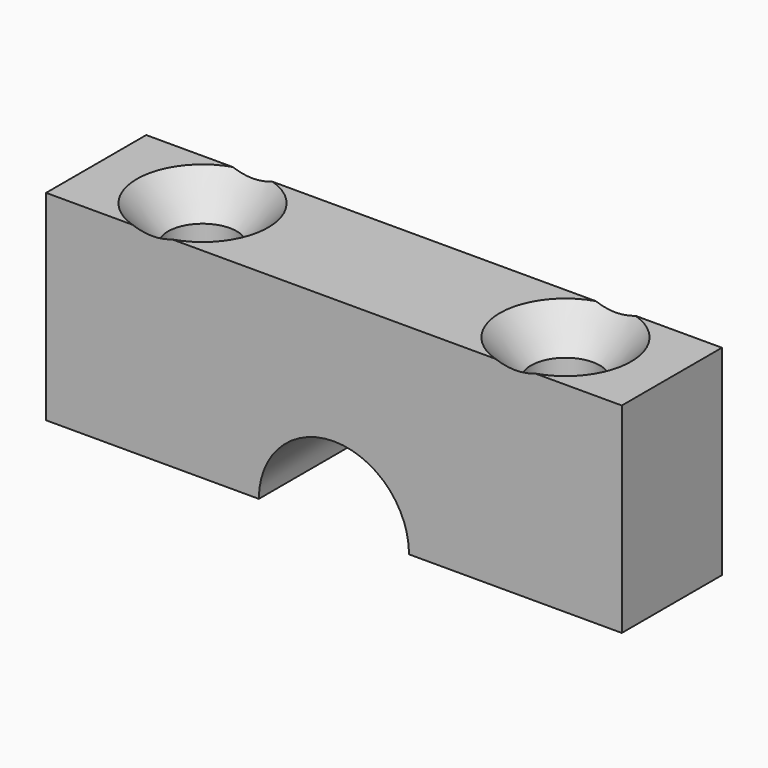
from build123d import *

# Parameters (mm, degrees)
F1_DEPTH       = 25.4
F2_D           = 8.7376
F2_DEPTH       = 29.6333418
F2_CSINK_D     = 16.6624
F2_CSINK_ANGLE = 82
F2_TIP         = 2.6250398724
F4_D           = 19.05


# Not quite as in the source:
# - a feature names something its author has since deleted; it is built from what else it names


with BuildPart() as f1:
    # F0 (on Top) → F1 (new body)
    with BuildSketch(Plane.XY):
        Polygon((36.5125, -7.9375), (36.5125, 7.9375), (0, 7.9375), (-36.5125, 7.9375), (-36.5125, -7.9375), align=None)
    extrude(amount=-F1_DEPTH)

    # F2
    with Locations(Plane.XY):
        with Locations((-23.01875, 0), (23.01875, 0)):
            CounterSinkHole(F2_D / 2, F2_CSINK_D / 2, depth=F2_DEPTH, counter_sink_angle=F2_CSINK_ANGLE)
            with Locations((0, 0, -(F2_DEPTH + F2_TIP / 2))):  # 118° drill point
                Cone(0, F2_D / 2, F2_TIP, mode=Mode.SUBTRACT)

    # F4 (through all)
    with Locations(Plane.XZ.offset(7.9375)):
        with Locations((0, -25.4)):
            Hole(F4_D / 2)


solid = f1.part
